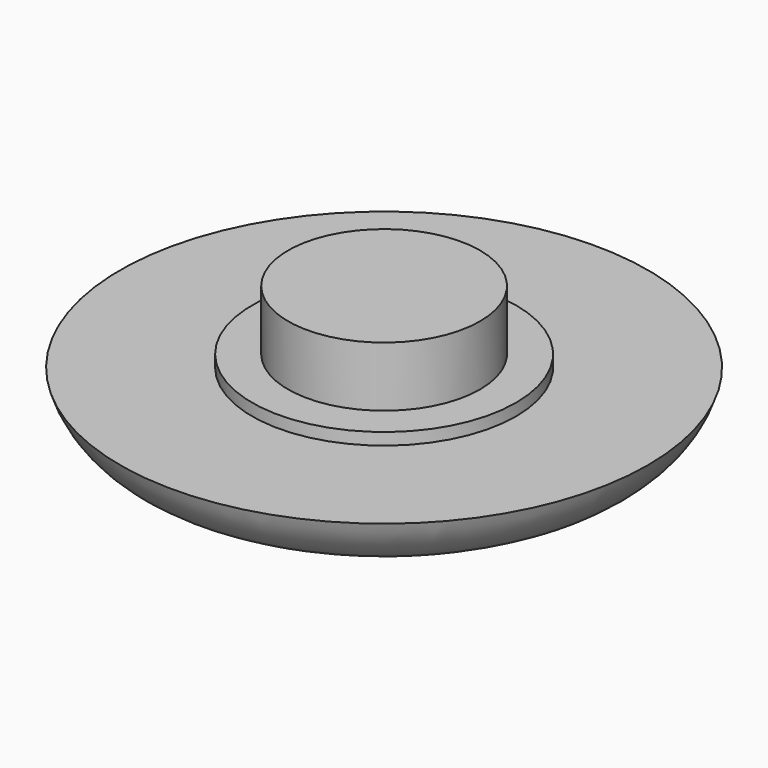
from build123d import *

# Parameters (mm, degrees)
F0_R         = 11
F0_R_2       = 5.5
F1_DEPTH     = 2.5
F0_R_3       = 4
F2_DEPTH     = 3
F3_DEPTH     = 5.5
F6_TEXT_SIZE = 4.6056071936
F7_DEPTH     = 1


# Not quite as in the source:
# - a fillet or chamfer that OpenCascade refuses, or shapes differently, is made with other operations: its cross-section is extruded or revolved along the edge and cut away or added
# - Text() gives the source's letters only with a copy of the font that has no kerning and outlines rounded to 1/6400 em; it was checked with that copy


with BuildPart() as f1:
    # F0 (on Top) → F1 (new body)
    with BuildSketch(Plane.XY):
        Circle(F0_R)
        Circle(F0_R_2, mode=Mode.SUBTRACT)
    extrude(amount=F1_DEPTH)

    # F0 (on Top) → F2 (join, through all)
    with BuildSketch(Plane.XY):
        Circle(F0_R_2)
        Circle(F0_R_3, mode=Mode.SUBTRACT)
    extrude(amount=F2_DEPTH)

    # F0 (on Top) → F3 (join, through all)
    with BuildSketch(Plane.XY):
        Circle(F0_R_3)
    extrude(amount=F3_DEPTH)

    # F4: fillet of radius 3.5 on 1 edges, made by hand

    # F4_s1 → F4_t2 (revolve, cut)
    with BuildSketch(Plane.XZ):
        with BuildLine():
            ThreePointArc((11, 2.5), (9.7375481001, 0.6937569599), (7.6458980338, 0))
            Line((7.6458980338, 0), (11, 0))
            Line((11, 0), (11, 2.5))
        make_face()
    revolve(axis=Axis((0, 0, 0), (0, 0, 1)), mode=Mode.SUBTRACT)

    # F6 (on face) → F7 (cut)
    with BuildSketch(Plane(origin=(0, 0, 0), x_dir=(1, 0, 0), z_dir=(0, 0, -1))):
        with Locations((-7.4639621582, -1.6580185897)):
            Text('DWITT', F6_TEXT_SIZE, font='Open Sans', font_style=FontStyle.BOLD, text_align=(TextAlign.LEFT, TextAlign.BOTTOM))
    extrude(amount=-F7_DEPTH, mode=Mode.SUBTRACT)


solid = f1.part
